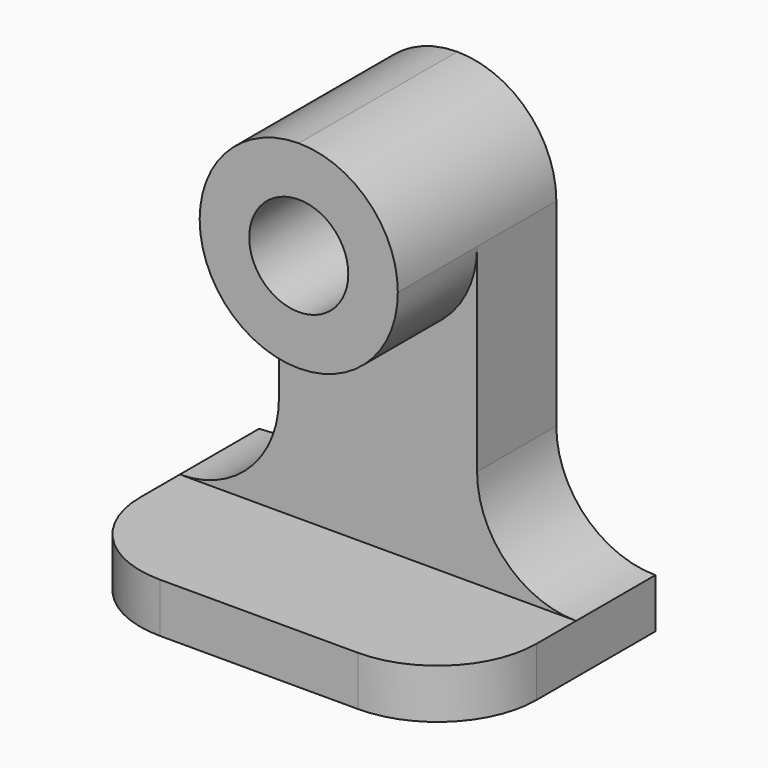
from build123d import *

# Parameters (mm, degrees)
F1_DEPTH  = 31.75
F2_R      = 6.35
F3_DEPTH  = 31.75
F5_DEPTH  = 31.75
F7_DEPTH  = 19.05
F8_DEPTH  = 6.35
F9_W      = 12.7
F9_H      = 12.7
F10_DEPTH = 31.75
F11_W     = 12.7
F11_H     = 12.7
F12_DEPTH = 19.05
F14_DEPTH = 12.7
F15_W     = 12.7
F15_H     = 12.7
F16_DEPTH = 12.7
F18_DEPTH = 12.7
F19_R     = 1.5875
F20_DEPTH = 12.7
F22_DEPTH = 6.35


# Not quite as in the source:
# - a feature names something its author has since deleted; it is built from what else it names


with BuildPart() as f1:
    # F0 (on Front) → F1 (new body)
    with BuildSketch(Plane.XZ):
        Polygon((-9.6981803781, 6.35), (-22.3981803781, 6.35), (-22.3981803781, 0), (28.4018196219, 0), (28.4018196219, 6.35), (15.7018196219, 6.35), (15.7018196219, 57.15), (-9.6981803781, 57.15), align=None)
    extrude(amount=F1_DEPTH)

    # F2 (on face) → F3 (cut)
    with BuildSketch(Plane.XZ.offset(31.75)):
        with Locations((3.0018196219, 44.45)):
            Circle(F2_R)
    extrude(amount=-F3_DEPTH, mode=Mode.SUBTRACT)

    # F4 (on face) → F5 (cut)
    with BuildSketch(Plane.XZ.offset(31.75)):
        with BuildLine():
            ThreePointArc((-9.6981803781, 44.45), (-5.9784365163, 53.4302561039), (3.0018195733, 57.15))
            Line((3.0018195733, 57.15), (-9.6981803781, 57.15))
            Line((-9.6981803781, 57.15), (-9.6981803781, 44.45))
        make_face()
        with BuildLine():
            ThreePointArc((3.0018195733, 57.15), (11.9820757258, 53.4302561383), (15.7018196219, 44.45))
            Line((15.7018196219, 44.45), (15.7018196219, 57.15))
            Line((15.7018196219, 57.15), (3.0018195733, 57.15))
        make_face()
    extrude(amount=-F5_DEPTH, mode=Mode.SUBTRACT)

    # F6 (on face) → F7 (cut)
    with BuildSketch(Plane.XZ.offset(31.75)):
        with BuildLine():
            Line((15.7018196219, 6.35), (15.7018196219, 44.45))
            ThreePointArc((15.7018196219, 44.45), (3.0018196219, 31.75), (-9.6981803781, 44.45))
            Line((-9.6981803781, 44.45), (-9.6981803781, 6.35))
            Line((-9.6981803781, 6.35), (15.7018196219, 6.35))
        make_face()
    extrude(amount=-F7_DEPTH, mode=Mode.SUBTRACT)

    # F8 (cut): a face of the model
    f8_faces = [f1.faces().sort_by_distance(p)[0] for p in [
        (15.3426093771, -31.75, 44.45),
    ]]
    extrude(f8_faces, amount=-F8_DEPTH, mode=Mode.SUBTRACT)

    # F9 (on face) → F10 (join)
    with BuildSketch(Plane.XZ.offset(31.75)):
        with Locations((-16.0481803781, 12.7)):
            Rectangle(F9_W, F9_H)
    extrude(amount=-F10_DEPTH)

    # F11 (on face) → F12 (cut)
    with BuildSketch(Plane.XZ.offset(31.75)):
        with Locations((-16.0481803781, 12.7)):
            Rectangle(F11_W, F11_H)
    extrude(amount=-F12_DEPTH, mode=Mode.SUBTRACT)

    # F13 (on face) → F14 (cut)
    with BuildSketch(Plane.XZ.offset(12.7)):
        with BuildLine():
            Line((-22.3981803781, 19.05), (-22.3981803781, 6.35))
            ThreePointArc((-22.3981803781, 6.35), (-13.417924257, 10.0697438789), (-9.6981803781, 19.05))
            Line((-9.6981803781, 19.05), (-22.3981803781, 19.05))
        make_face()
    extrude(amount=-F14_DEPTH, mode=Mode.SUBTRACT)

    # F15 (on face) → F16 (join)
    with BuildSketch(Plane.XZ.offset(12.7)):
        with Locations((22.0518196219, 12.7)):
            Rectangle(F15_W, F15_H)
    extrude(amount=-F16_DEPTH)

    # F17 (on face) → F18 (cut)
    with BuildSketch(Plane.XZ.offset(12.7)):
        with BuildLine():
            Line((28.4018196219, 19.05), (15.7018196219, 19.05))
            ThreePointArc((15.7018196219, 19.05), (19.4215635009, 10.0697438789), (28.4018196219, 6.35))
            Line((28.4018196219, 6.35), (28.4018196219, 19.05))
        make_face()
    extrude(amount=-F18_DEPTH, mode=Mode.SUBTRACT)

    # F19 (on Top) → F20 (cut)
    with BuildSketch(Plane.XY):
        with Locations((-12.8731803781, -22.225)):
            Circle(F19_R)
        with Locations((18.8768196219, -22.225)):
            Circle(F19_R)
    extrude(amount=-F20_DEPTH, mode=Mode.SUBTRACT)

    # F21 (on face) → F22 (cut)
    with BuildSketch(Plane.XY.offset(6.35)):
        with BuildLine():
            ThreePointArc((-9.6981803781, -31.75), (-18.6784364991, -28.0302561211), (-22.3981803781, -19.05))
            Line((-22.3981803781, -19.05), (-22.3981803781, -31.75))
            Line((-22.3981803781, -31.75), (-9.6981803781, -31.75))
        make_face()
        with BuildLine():
            ThreePointArc((28.4018196219, -19.05), (24.682075743, -28.0302561211), (15.7018196219, -31.75))
            Line((15.7018196219, -31.75), (28.4018196219, -31.75))
            Line((28.4018196219, -31.75), (28.4018196219, -19.05))
        make_face()
    extrude(amount=-F22_DEPTH, mode=Mode.SUBTRACT)


solid = f1.part
